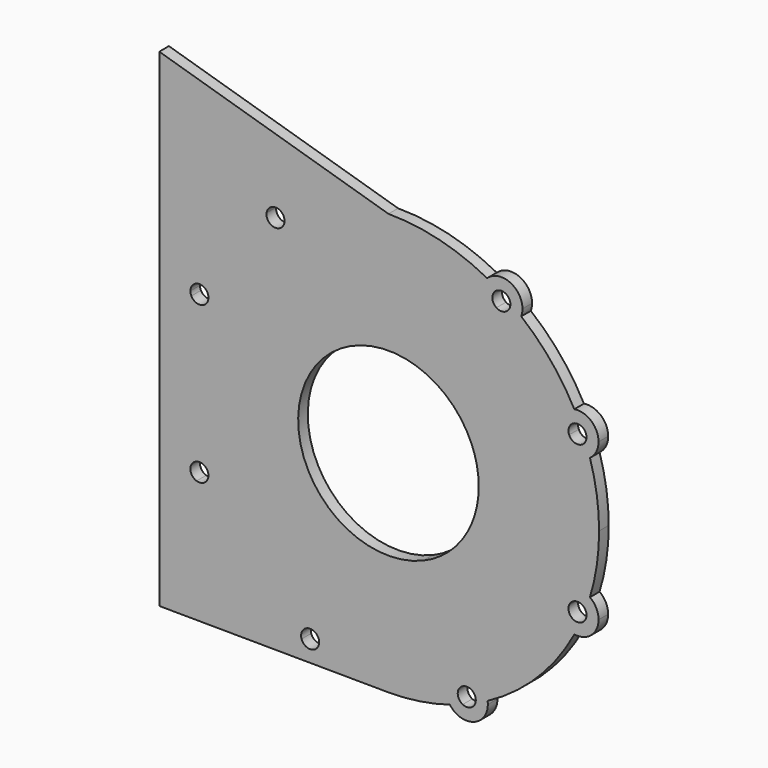
from build123d import *

# Parameters (mm, degrees)
F1_DEPTH = 6


with BuildPart() as f1:
    # F0 (on Front) → F1 (new body)
    with BuildSketch(Plane.XZ):
        with BuildLine():
            ThreePointArc((100.4510831721, -30.5708993907), (103.8565446495, -15.4537417302), (105, 0))
            ThreePointArc((105, 0), (103.8565446495, 15.4537417302), (100.4510831721, 30.5708993907))
            ThreePointArc((100.4510831721, 30.5708993907), (91.4115955865, 28.9206312082), (84.5349772248, 35.0155340614))
            Line((84.5349772248, 35.0155340614), (41.574578963, 17.2207544564))
            ThreePointArc((41.574578963, 17.2207544564), (44.1353376181, 8.7790644907), (45, 0))
            ThreePointArc((45, 0), (44.1353376181, -8.7790644907), (41.574578963, -17.2207544564))
            Line((41.574578963, -17.2207544564), (84.5349772248, -35.0155340614))
            ThreePointArc((84.5349772248, -35.0155340614), (91.4115955865, -28.9206312082), (100.4510831721, -30.5708993907))
        make_face()
        with BuildLine():
            ThreePointArc((84.5349772248, 35.0155340614), (91.4115955865, 28.9206312082), (100.4510831721, 30.5708993907))
            ThreePointArc((100.4510831721, 30.5708993907), (99.407070598, 33.8117481819), (98.2585290039, 37.0170430746))
            ThreePointArc((98.2585290039, 37.0170430746), (94.0737613555, 34.5366252803), (90.0782544199, 37.3116346556))
            Line((90.0782544199, 37.3116346556), (84.5349772248, 35.0155340614))
        make_face()
        with BuildLine():
            ThreePointArc((98.2585290039, 37.0170430746), (99.407070598, 33.8117481819), (100.4510831721, 30.5708993907))
            ThreePointArc((100.4510831721, 30.5708993907), (103.6035133918, 34.2908941649), (104.7357123162, 39.0337101012))
            ThreePointArc((104.7357123162, 39.0337101012), (101.075434913, 47.0004029407), (92.6465323546, 49.4127518224))
            ThreePointArc((92.6465323546, 49.4127518224), (94.199930141, 46.3828972946), (95.6542743456, 43.3042699906))
            ThreePointArc((95.6542743456, 43.3042699906), (97.8849265557, 41.6668138656), (98.7357123162, 39.0337101012))
            ThreePointArc((98.7357123162, 39.0337101012), (98.6147918481, 37.997533257), (98.2585290039, 37.0170430746))
        make_face()
        with BuildLine():
            ThreePointArc((104.7357123162, -39.0337101012), (103.6035133918, -34.2908941649), (100.4510831721, -30.5708993907))
            ThreePointArc((100.4510831721, -30.5708993907), (99.407070598, -33.8117481819), (98.2585290039, -37.0170430746))
            ThreePointArc((98.2585290039, -37.0170430746), (98.6147918481, -37.997533257), (98.7357123162, -39.0337101012))
            ThreePointArc((98.7357123162, -39.0337101012), (97.8849265557, -41.6668138656), (95.6542743456, -43.3042699906))
            ThreePointArc((95.6542743456, -43.3042699906), (94.199930141, -46.3828972946), (92.6465323546, -49.4127518224))
            ThreePointArc((92.6465323546, -49.4127518224), (101.075434913, -47.0004029407), (104.7357123162, -39.0337101012))
        make_face()
        with BuildLine():
            ThreePointArc((98.2585290039, -37.0170430746), (99.407070598, -33.8117481819), (100.4510831721, -30.5708993907))
            ThreePointArc((100.4510831721, -30.5708993907), (91.4115955865, -28.9206312082), (84.5349772248, -35.0155340614))
            Line((84.5349772248, -35.0155340614), (90.0782544199, -37.3116346556))
            ThreePointArc((90.0782544199, -37.3116346556), (94.0737613555, -34.5366252803), (98.2585290039, -37.0170430746))
        make_face()
        with BuildLine():
            ThreePointArc((92.6465323546, 49.4127518224), (85.0877335618, 44.1877846748), (84.5349772248, 35.0155340614))
            Line((84.5349772248, 35.0155340614), (90.0782544199, 37.3116346556))
            ThreePointArc((90.0782544199, 37.3116346556), (90.9412765212, 42.0991126512), (95.6542743456, 43.3042699906))
            ThreePointArc((95.6542743456, 43.3042699906), (94.199930141, 46.3828972946), (92.6465323546, 49.4127518224))
        make_face()
        with BuildLine():
            Line((41.574578963, 17.2207544564), (84.5349772248, 35.0155340614))
            ThreePointArc((84.5349772248, 35.0155340614), (85.0877335618, 44.1877846748), (92.6465323546, 49.4127518224))
            ThreePointArc((92.6465323546, 49.4127518224), (81.0205812557, 66.7882131292), (66.1826921615, 81.5159570774))
            ThreePointArc((66.1826921615, 81.5159570774), (59.6114355729, 75.0930054405), (50.5022341561, 76.3005527191))
            Line((50.5022341561, 76.3005527191), (24.837164339, 37.524861993))
            ThreePointArc((24.837164339, 37.524861993), (34.7231062524, 28.6235199125), (41.574578963, 17.2207544564))
        make_face()
        with BuildLine():
            ThreePointArc((92.6465323546, -49.4127518224), (85.0877335618, -44.1877846748), (84.5349772248, -35.0155340614))
            Line((84.5349772248, -35.0155340614), (41.574578963, -17.2207544564))
            ThreePointArc((41.574578963, -17.2207544564), (31.8198051534, -31.8198051534), (17.2207544564, -41.574578963))
            Line((17.2207544564, -41.574578963), (35.0155340614, -84.5349772248))
            ThreePointArc((35.0155340614, -84.5349772248), (44.1877846748, -85.0877335618), (49.4127518224, -92.6465323546))
            ThreePointArc((49.4127518224, -92.6465323546), (74.2462120246, -74.2462120246), (92.6465323546, -49.4127518224))
        make_face()
        with BuildLine():
            Line((90.0782544199, -37.3116346556), (84.5349772248, -35.0155340614))
            ThreePointArc((84.5349772248, -35.0155340614), (85.0877335618, -44.1877846748), (92.6465323546, -49.4127518224))
            ThreePointArc((92.6465323546, -49.4127518224), (94.199930141, -46.3828972946), (95.6542743456, -43.3042699906))
            ThreePointArc((95.6542743456, -43.3042699906), (90.9412765212, -42.0991126512), (90.0782544199, -37.3116346556))
        make_face()
        with BuildLine():
            ThreePointArc((17.2207544564, -41.574578963), (-44.7928289265, 4.3130588634), (24.837164339, 37.524861993))
            Line((24.837164339, 37.524861993), (50.5022341561, 76.3005527191))
            ThreePointArc((50.5022341561, 76.3005527191), (45.831432476, 84.2137905236), (49.1761961289, 92.772311248))
            ThreePointArc((49.1761961289, 92.772311248), (25.3368044449, 101.8972342143), (0, 105))
            ThreePointArc((0, 105), (-25.3368044449, 101.8972342143), (-49.1761961289, 92.772311248))
            ThreePointArc((-49.1761961289, 92.772311248), (-46.6792448947, 89.2679775332), (-45.7975725018, 85.0563538509))
            ThreePointArc((-45.7975725018, 85.0563538509), (-54.5008750352, 74.7112159488), (-66.1826921615, 81.5159570774))
            ThreePointArc((-66.1826921615, 81.5159570774), (-81.0205812557, 66.7882131292), (-92.6465323546, 49.4127518224))
            ThreePointArc((-92.6465323546, 49.4127518224), (-86.2690194767, 45.8734326981), (-83.7357123162, 39.0337101012))
            ThreePointArc((-83.7357123162, 39.0337101012), (-89.4928963798, 29.6659090256), (-100.4510831721, 30.5708993907))
            ThreePointArc((-100.4510831721, 30.5708993907), (-105, 0), (-100.4510831721, -30.5708993907))
            ThreePointArc((-100.4510831721, -30.5708993907), (-89.4928963798, -29.6659090255), (-83.7357123162, -39.0337101012))
            ThreePointArc((-83.7357123162, -39.0337101012), (-86.2690194767, -45.8734326981), (-92.6465323546, -49.4127518224))
            ThreePointArc((-92.6465323546, -49.4127518224), (-74.2462120246, -74.2462120246), (-49.4127518224, -92.6465323546))
            ThreePointArc((-49.4127518224, -92.6465323546), (-38.2368218005, -83.7659955561), (-28.5337101012, -94.2357123162))
            ThreePointArc((-28.5337101012, -94.2357123162), (-29.0559971253, -97.506070671), (-30.5708993907, -100.4510831721))
            ThreePointArc((-30.5708993907, -100.4510831721), (-16.1559201029, -103.7496325084), (-1.4205010638, -104.9903908781))
            Line((-1.4205010638, -104.9903908781), (0, -105))
            ThreePointArc((0, -105), (15.4537417302, -103.8565446495), (30.5708993907, -100.4510831721))
            ThreePointArc((30.5708993907, -100.4510831721), (28.9206312082, -91.4115955865), (35.0155340614, -84.5349772248))
            Line((35.0155340614, -84.5349772248), (17.2207544564, -41.574578963))
        make_face()
        with BuildLine():
            ThreePointArc((50.5022341561, 76.3005527191), (59.6114355729, 75.0930054405), (66.1826921615, 81.5159570774))
            ThreePointArc((66.1826921615, 81.5159570774), (63.5049068662, 83.6189380698), (60.7603445735, 85.6339916582))
            ThreePointArc((60.7603445735, 85.6339916582), (60.7882558754, 85.3457719546), (60.7975725018, 85.0563538509))
            ThreePointArc((60.7975725018, 85.0563538509), (58.4275110042, 81.0923455289), (53.8138560679, 81.3038676515))
            Line((53.8138560679, 81.3038676515), (50.5022341561, 76.3005527191))
        make_face()
        with BuildLine():
            ThreePointArc((60.7603445735, 85.6339916582), (63.5049068662, 83.6189380698), (66.1826921615, 81.5159570774))
            ThreePointArc((66.1826921615, 81.5159570774), (66.6427104039, 83.2596563842), (66.7975725018, 85.0563538509))
            ThreePointArc((66.7975725018, 85.0563538509), (60.5091961842, 94.674681458), (49.1761961289, 92.772311248))
            ThreePointArc((49.1761961289, 92.772311248), (52.1582944094, 91.1290970234), (55.0855469393, 89.390058275))
            ThreePointArc((55.0855469393, 89.390058275), (58.7812889357, 88.8088400502), (60.7603445735, 85.6339916582))
        make_face()
        with BuildLine():
            ThreePointArc((49.5337101012, -94.2357123162), (49.5034268613, -93.4388240154), (49.4127518224, -92.6465323546))
            ThreePointArc((49.4127518224, -92.6465323546), (46.3828972946, -94.199930141), (43.3042699906, -95.6542743456))
            ThreePointArc((43.3042699906, -95.6542743456), (40.7557855469, -98.3931702125), (37.0170430746, -98.2585290039))
            ThreePointArc((37.0170430746, -98.2585290039), (33.8117481819, -99.407070598), (30.5708993907, -100.4510831721))
            ThreePointArc((30.5708993907, -100.4510831721), (42.3040684561, -104.2134252921), (49.5337101012, -94.2357123162))
        make_face()
        with BuildLine():
            ThreePointArc((43.3042699906, -95.6542743456), (46.3828972946, -94.199930141), (49.4127518224, -92.6465323546))
            ThreePointArc((49.4127518224, -92.6465323546), (44.1877846748, -85.0877335618), (35.0155340614, -84.5349772248))
            Line((35.0155340614, -84.5349772248), (37.3116346556, -90.0782544199))
            ThreePointArc((37.3116346556, -90.0782544199), (41.5337761498, -90.4940990608), (43.5337101012, -94.2357123162))
            ThreePointArc((43.5337101012, -94.2357123162), (43.4759797634, -94.9542109236), (43.3042699906, -95.6542743456))
        make_face()
        with BuildLine():
            ThreePointArc((49.1761961289, 92.772311248), (45.831432476, 84.2137905236), (50.5022341561, 76.3005527191))
            Line((50.5022341561, 76.3005527191), (53.8138560679, 81.3038676515))
            ThreePointArc((53.8138560679, 81.3038676515), (51.8522100953, 85.7554626223), (55.0855469393, 89.390058275))
            ThreePointArc((55.0855469393, 89.390058275), (52.1582944094, 91.1290970234), (49.1761961289, 92.772311248))
        make_face()
        with BuildLine():
            Line((37.3116346556, -90.0782544199), (35.0155340614, -84.5349772248))
            ThreePointArc((35.0155340614, -84.5349772248), (28.9206312082, -91.4115955865), (30.5708993907, -100.4510831721))
            ThreePointArc((30.5708993907, -100.4510831721), (33.8117481819, -99.407070598), (37.0170430746, -98.2585290039))
            ThreePointArc((37.0170430746, -98.2585290039), (34.5366252803, -94.0737613555), (37.3116346556, -90.0782544199))
        make_face()
        with BuildLine():
            ThreePointArc((-49.1761961289, 92.772311248), (-25.3368044449, 101.8972342143), (0, 105))
            Line((0, 105), (-114.2357123162, 139.0337101012))
            Line((-114.2357123162, 139.0337101012), (-114.2357123162, 39.0337101012))
            Line((-114.2357123162, 39.0337101012), (-104.7357123162, 39.0337101012))
            ThreePointArc((-104.7357123162, 39.0337101012), (-101.075434913, 47.0004029407), (-92.6465323546, 49.4127518224))
            ThreePointArc((-92.6465323546, 49.4127518224), (-81.0205812557, 66.7882131292), (-66.1826921615, 81.5159570774))
            ThreePointArc((-66.1826921615, 81.5159570774), (-62.0929108476, 93.8121549826), (-49.1761961289, 92.772311248))
        make_face()
        with BuildLine():
            ThreePointArc((-45.7975725018, 85.0563538509), (-46.6792448947, 89.2679775332), (-49.1761961289, 92.772311248))
            ThreePointArc((-49.1761961289, 92.772311248), (-52.1582944094, 91.1290970234), (-55.0855469393, 89.390058275))
            ThreePointArc((-55.0855469393, 89.390058275), (-52.7125958609, 87.7762697474), (-51.7975725018, 85.0563538509))
            ThreePointArc((-51.7975725018, 85.0563538509), (-56.5869906056, 80.5656704773), (-60.7603445735, 85.6339916582))
            ThreePointArc((-60.7603445735, 85.6339916582), (-63.5049068662, 83.6189380698), (-66.1826921615, 81.5159570774))
            ThreePointArc((-66.1826921615, 81.5159570774), (-54.5008750352, 74.7112159488), (-45.7975725018, 85.0563538509))
        make_face()
        with BuildLine():
            ThreePointArc((-55.0855469393, 89.390058275), (-52.1582944094, 91.1290970234), (-49.1761961289, 92.772311248))
            ThreePointArc((-49.1761961289, 92.772311248), (-62.0929108476, 93.8121549826), (-66.1826921615, 81.5159570774))
            ThreePointArc((-66.1826921615, 81.5159570774), (-63.5049068662, 83.6189380698), (-60.7603445735, 85.6339916582))
            ThreePointArc((-60.7603445735, 85.6339916582), (-58.7812889357, 88.8088400502), (-55.0855469393, 89.390058275))
        make_face()
        with BuildLine():
            Line((-39.1047365684, -104.7354720868), (-1.4205010638, -104.9903908781))
            ThreePointArc((-1.4205010638, -104.9903908781), (-16.1559201029, -103.7496325084), (-30.5708993907, -100.4510831721))
            ThreePointArc((-30.5708993907, -100.4510831721), (-34.3226053699, -103.6195011144), (-39.1047365684, -104.7354720868))
        make_face()
        with BuildLine():
            Line((-104.7357123162, 39.0337101012), (-114.2357123162, 39.0337101012))
            Line((-114.2357123162, 39.0337101012), (-114.2357123162, -104.2272410647))
            Line((-114.2357123162, -104.2272410647), (-39.1047365684, -104.7354720868))
            ThreePointArc((-39.1047365684, -104.7354720868), (-47.0234909022, -101.0484505874), (-49.4127518224, -92.6465323546))
            ThreePointArc((-49.4127518224, -92.6465323546), (-74.2462120246, -74.2462120246), (-92.6465323546, -49.4127518224))
            ThreePointArc((-92.6465323546, -49.4127518224), (-103.9364474075, -43.0518861411), (-100.4510831721, -30.5708993907))
            ThreePointArc((-100.4510831721, -30.5708993907), (-105, 0), (-100.4510831721, 30.5708993907))
            ThreePointArc((-100.4510831721, 30.5708993907), (-103.6035133918, 34.2908941649), (-104.7357123162, 39.0337101012))
        make_face()
        with BuildLine():
            ThreePointArc((-39.1047365684, -104.7354720868), (-34.3226053699, -103.6195011144), (-30.5708993907, -100.4510831721))
            ThreePointArc((-30.5708993907, -100.4510831721), (-33.8117481819, -99.407070598), (-37.0170430746, -98.2585290039))
            ThreePointArc((-37.0170430746, -98.2585290039), (-40.7557855469, -98.3931702125), (-43.3042699906, -95.6542743456))
            ThreePointArc((-43.3042699906, -95.6542743456), (-46.3828972946, -94.199930141), (-49.4127518224, -92.6465323546))
            ThreePointArc((-49.4127518224, -92.6465323546), (-47.0234909022, -101.0484505874), (-39.1047365684, -104.7354720868))
        make_face()
        with BuildLine():
            ThreePointArc((-37.0170430746, -98.2585290039), (-33.8117481819, -99.407070598), (-30.5708993907, -100.4510831721))
            ThreePointArc((-30.5708993907, -100.4510831721), (-29.0559971253, -97.506070671), (-28.5337101012, -94.2357123162))
            ThreePointArc((-28.5337101012, -94.2357123162), (-38.2368218005, -83.7659955561), (-49.4127518224, -92.6465323546))
            ThreePointArc((-49.4127518224, -92.6465323546), (-46.3828972946, -94.199930141), (-43.3042699906, -95.6542743456))
            ThreePointArc((-43.3042699906, -95.6542743456), (-39.7522087087, -89.793442654), (-34.5337101012, -94.2357123162))
            ThreePointArc((-34.5337101012, -94.2357123162), (-35.2045455958, -96.5995014755), (-37.0170430746, -98.2585290039))
        make_face()
        with BuildLine():
            ThreePointArc((-83.7357123162, 39.0337101012), (-86.2690194767, 45.8734326981), (-92.6465323546, 49.4127518224))
            ThreePointArc((-92.6465323546, 49.4127518224), (-94.199930141, 46.3828972946), (-95.6542743456, 43.3042699906))
            ThreePointArc((-95.6542743456, 43.3042699906), (-91.6026085518, 42.6829243408), (-89.7357123162, 39.0337101012))
            ThreePointArc((-89.7357123162, 39.0337101012), (-93.1995354719, 34.6546305692), (-98.2585290039, 37.0170430746))
            ThreePointArc((-98.2585290039, 37.0170430746), (-99.407070598, 33.8117481819), (-100.4510831721, 30.5708993907))
            ThreePointArc((-100.4510831721, 30.5708993907), (-89.4928963798, 29.6659090256), (-83.7357123162, 39.0337101012))
        make_face()
        with BuildLine():
            ThreePointArc((-95.6542743456, 43.3042699906), (-94.199930141, 46.3828972946), (-92.6465323546, 49.4127518224))
            ThreePointArc((-92.6465323546, 49.4127518224), (-101.075434913, 47.0004029407), (-104.7357123162, 39.0337101012))
            Line((-104.7357123162, 39.0337101012), (-98.7357123162, 39.0337101012))
            ThreePointArc((-98.7357123162, 39.0337101012), (-97.8849265557, 41.6668138656), (-95.6542743456, 43.3042699906))
        make_face()
        with BuildLine():
            Line((-98.7357123162, 39.0337101012), (-104.7357123162, 39.0337101012))
            ThreePointArc((-104.7357123162, 39.0337101012), (-103.6035133918, 34.2908941649), (-100.4510831721, 30.5708993907))
            ThreePointArc((-100.4510831721, 30.5708993907), (-99.407070598, 33.8117481819), (-98.2585290039, 37.0170430746))
            ThreePointArc((-98.2585290039, 37.0170430746), (-98.6147918481, 37.997533257), (-98.7357123162, 39.0337101012))
        make_face()
        with BuildLine():
            ThreePointArc((-100.4510831721, -30.5708993907), (-103.9364474075, -43.0518861411), (-92.6465323546, -49.4127518224))
            ThreePointArc((-92.6465323546, -49.4127518224), (-94.199930141, -46.3828972946), (-95.6542743456, -43.3042699906))
            ThreePointArc((-95.6542743456, -43.3042699906), (-98.3931702125, -40.7557855469), (-98.2585290039, -37.0170430746))
            ThreePointArc((-98.2585290039, -37.0170430746), (-99.407070598, -33.8117481819), (-100.4510831721, -30.5708993907))
        make_face()
        with BuildLine():
            ThreePointArc((-95.6542743456, -43.3042699906), (-94.199930141, -46.3828972946), (-92.6465323546, -49.4127518224))
            ThreePointArc((-92.6465323546, -49.4127518224), (-86.2690194767, -45.8734326981), (-83.7357123162, -39.0337101012))
            ThreePointArc((-83.7357123162, -39.0337101012), (-89.4928963798, -29.6659090255), (-100.4510831721, -30.5708993907))
            ThreePointArc((-100.4510831721, -30.5708993907), (-99.407070598, -33.8117481819), (-98.2585290039, -37.0170430746))
            ThreePointArc((-98.2585290039, -37.0170430746), (-93.1995354719, -34.6546305692), (-89.7357123162, -39.0337101012))
            ThreePointArc((-89.7357123162, -39.0337101012), (-91.6026085518, -42.6829243408), (-95.6542743456, -43.3042699906))
        make_face()
    extrude(amount=F1_DEPTH)


solid = f1.part
